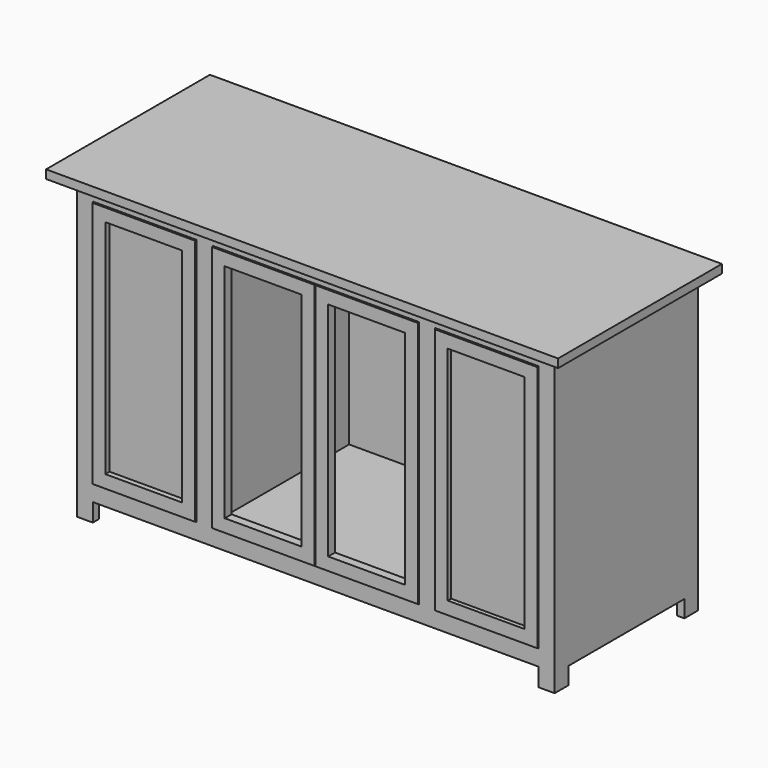
from build123d import *

# Parameters (mm, degrees)
F0_W      = 1524
F0_H      = 609.6
F1_DEPTH  = 25.4
F2_W      = 22.225
F2_H      = 511.175
F3_DEPTH  = 889
F2_W_2    = 19.05
F2_H_2    = 504.825
F4_DEPTH  = 787.4
F6_W      = 1377.95
F6_H      = 504.825
F7_DEPTH  = 12.7
F9_W      = 47.625
F9_H      = 739.775
F10_DEPTH = 22.225
F11_W     = 228.6
F11_H     = 38.1
F12_DEPTH = 25.4
F13_W     = 1377.95
F13_H     = 6.35
F14_DEPTH = 800.1
F15_W     = 228.6
F15_H     = 9.525
F16_DEPTH = 660.4
F15_H_2   = 3.175
F17_DEPTH = 660.4
F18_W     = 431.8
F18_H     = 50.8
F19_DEPTH = 1473.201


with BuildPart() as f1:
    # F0 (on Top) → F1 (new body)
    with BuildSketch(Plane.XY):
        Rectangle(F0_W, F0_H)
    extrude(amount=F1_DEPTH)

    # F2 (on face) → F3 (join)
    with BuildSketch(Plane(origin=(0, 0, 0), x_dir=(1, 0, 0), z_dir=(0, 0, -1))):
        with Locations((-700.0875, -23.8125)):
            Rectangle(F2_W, F2_H)
        with Locations((700.0875, -23.8125)):
            Rectangle(F2_W, F2_H)
    extrude(amount=F3_DEPTH)

    # F2 (on face) → F4 (join)
    with BuildSketch(Plane(origin=(0, 0, 0), x_dir=(1, 0, 0), z_dir=(0, 0, -1))):
        with Locations((-700.0875, -23.8125)):
            Rectangle(F2_W, F2_H)
        with Locations((700.0875, -23.8125)):
            Rectangle(F2_W, F2_H)
        with Locations((-331.7875, -20.6375)):
            Rectangle(F2_W_2, F2_H_2)
        with Locations((331.7875, -20.6375)):
            Rectangle(F2_W_2, F2_H_2)
    extrude(amount=F4_DEPTH)

    # F6 (on offset) → F7 (join)
    with BuildSketch(Plane(origin=(0, 0, -787.4), x_dir=(1, 0, 0), z_dir=(0, 0, -1))):
        with Locations((0, -20.6375)):
            Rectangle(F6_W, F6_H)
    extrude(amount=F7_DEPTH)

    # F9 (on offset) → F10 (join)
    with BuildSketch(Plane.XZ.offset(231.775)):
        Polygon((-663.575, 0), (-711.2, 0), (-711.2, -889), (-663.575, -889), (-663.575, -835.025), (-663.575, -787.4), (-663.575, -47.625), align=None)
        Polygon((663.575, 0), (-663.575, 0), (-663.575, -47.625), (-355.6, -47.625), (-307.975, -47.625), (307.975, -47.625), (355.6, -47.625), (663.575, -47.625), align=None)
        Polygon((711.2, 0), (663.575, 0), (663.575, -47.625), (663.575, -787.4), (663.575, -835.025), (663.575, -889), (711.2, -889), align=None)
        Polygon((-355.6, -787.4), (-663.575, -787.4), (-663.575, -835.025), (663.575, -835.025), (663.575, -787.4), (355.6, -787.4), (307.975, -787.4), (-307.975, -787.4), align=None)
        with Locations((-331.7875, -417.5125)):
            Rectangle(F9_W, F9_H)
        with Locations((331.7875, -417.5125)):
            Rectangle(F9_W, F9_H)
    extrude(amount=F10_DEPTH)

    # F13 (on face) → F14 (join, through all)
    with BuildSketch(Plane(origin=(0, 0, 0), x_dir=(1, 0, 0), z_dir=(0, 0, -1))):
        with Locations((0, -276.225)):
            Rectangle(F13_W, F13_H)
    extrude(amount=F14_DEPTH)

    # F18 (on face) → F19 (cut, through all)
    with BuildSketch(Plane.YZ.offset(711.2)):
        with Locations((12.7, -863.6)):
            Rectangle(F18_W, F18_H)
    extrude(amount=-F19_DEPTH, mode=Mode.SUBTRACT)


with BuildPart() as f12:
    # F11 (on offset) → F12 (new body)
    with BuildSketch(Plane.XZ.offset(231.775)):
        Polygon((-623.8875, -49.2125), (-661.9875, -49.2125), (-661.9875, -785.8125), (-623.8875, -785.8125), (-623.8875, -747.7125), (-623.8875, -87.3125), align=None)
        with Locations((-509.5875, -68.2625)):
            Rectangle(F11_W, F11_H)
        Polygon((-357.1875, -49.2125), (-395.2875, -49.2125), (-395.2875, -87.3125), (-395.2875, -747.7125), (-395.2875, -785.8125), (-357.1875, -785.8125), align=None)
        with Locations((-509.5875, -766.7625)):
            Rectangle(F11_W, F11_H)
    extrude(amount=F12_DEPTH)

    # F15 (on face) → F16 (join, through all)
    with BuildSketch(Plane.XY.offset(-747.7125)):
        with Locations((-509.5875, -236.5375)):
            Rectangle(F15_W, F15_H)
    extrude(amount=F16_DEPTH)


with BuildPart() as f12b:
    # F11 (on offset) → F12, piece 2 (new body)
    with BuildSketch(Plane.XZ.offset(231.775)):
        Polygon((357.1875, -785.8125), (395.2875, -785.8125), (395.2875, -747.7125), (395.2875, -87.3125), (395.2875, -49.2125), (357.1875, -49.2125), align=None)
        with Locations((509.5875, -766.7625)):
            Rectangle(F11_W, F11_H)
        Polygon((623.8875, -747.7125), (623.8875, -785.8125), (661.9875, -785.8125), (661.9875, -49.2125), (623.8875, -49.2125), (623.8875, -87.3125), align=None)
        with Locations((509.5875, -68.2625)):
            Rectangle(F11_W, F11_H)
    extrude(amount=F12_DEPTH)

    # F15 (on face) → F17 (join, through all)
    with BuildSketch(Plane.XY.offset(-747.7125)):
        with Locations((509.5875, -242.8875)):
            Rectangle(F15_W, F15_H_2)
    extrude(amount=F17_DEPTH)


with BuildPart() as f12c:
    # F11 (on offset) → F12, piece 3 (new body)
    with BuildSketch(Plane.XZ.offset(231.775)):
        Polygon((-268.2875, -49.2125), (-306.3875, -49.2125), (-306.3875, -785.8125), (-268.2875, -785.8125), (-268.2875, -747.7125), (-268.2875, -87.3125), align=None)
        with Locations((-153.9875, -68.2625)):
            Rectangle(F11_W, F11_H)
        Polygon((-1.5875, -49.2125), (-39.6875, -49.2125), (-39.6875, -87.3125), (-39.6875, -747.7125), (-39.6875, -785.8125), (-1.5875, -785.8125), align=None)
        with Locations((-153.9875, -766.7625)):
            Rectangle(F11_W, F11_H)
    extrude(amount=F12_DEPTH)


with BuildPart() as f12d:
    # F11 (on offset) → F12, piece 4 (new body)
    with BuildSketch(Plane.XZ.offset(231.775)):
        Polygon((306.3875, -785.8125), (306.3875, -49.2125), (268.2875, -49.2125), (268.2875, -87.3125), (268.2875, -747.7125), (268.2875, -785.8125), align=None)
        with Locations((153.9875, -68.2625)):
            Rectangle(F11_W, F11_H)
        Polygon((39.6875, -87.3125), (39.6875, -49.2125), (1.5875, -49.2125), (1.5875, -785.8125), (39.6875, -785.8125), (39.6875, -747.7125), align=None)
        with Locations((153.9875, -766.7625)):
            Rectangle(F11_W, F11_H)
    extrude(amount=F12_DEPTH)


solid = Compound([f1.part, f12.part, f12b.part, f12c.part, f12d.part])
